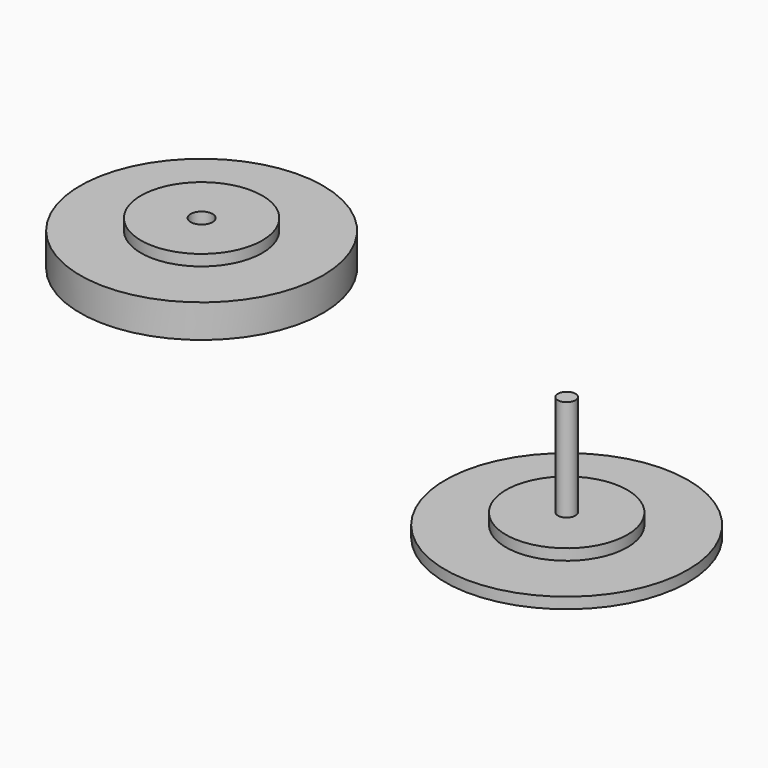
from build123d import *

# Parameters (mm, degrees)
F0_R      = 5.5
F1_DEPTH  = 0.5
F2_R      = 5.5
F3_DEPTH  = 0.5
F4_R      = 2.75
F5_DEPTH  = 1
F6_R      = 2.75
F7_DEPTH  = 1
F8_R      = 0.5
F9_DEPTH  = 0.7
F10_R     = 0.4
F11_DEPTH = 4.6
F13_DEPTH = 1


# Not quite as in the source:
# - the program builds the solid bodies; features that only make, move or delete a surface that nothing else refers to are left out


with BuildPart() as f1:
    # F0 (on Top) → F1 (new body)
    with BuildSketch(Plane.XY):
        with Locations((-49.2776818573, 41.9655069709)):
            Circle(F0_R)
    extrude(amount=F1_DEPTH)

    # F4 (on Top) → F5 (join)
    with BuildSketch(Plane.XY):
        with Locations((-49.2776595056, 41.9656410813)):
            Circle(F4_R)
    extrude(amount=F5_DEPTH)

    # F8 (on face) → F9 (cut)
    with BuildSketch(Plane.XY.offset(1)):
        with Locations((-49.2776595056, 41.9656410813)):
            Circle(F8_R)
    extrude(amount=-F9_DEPTH, mode=Mode.SUBTRACT)

    # F0 (on Top) → F13 (join)
    with BuildSketch(Plane.XY):
        with Locations((-49.2776818573, 41.9655069709)):
            Circle(F0_R)
    extrude(amount=-F13_DEPTH)


with BuildPart() as f3:
    # F2 (on Top) → F3 (new body)
    with BuildSketch(Plane.XY):
        with Locations((-25.1157227904, 32.4278958142)):
            Circle(F2_R)
    extrude(amount=F3_DEPTH)

    # F6 (on Top) → F7 (join)
    with BuildSketch(Plane.XY):
        with Locations((-25.1157619059, 32.4279852211)):
            Circle(F6_R)
    extrude(amount=F7_DEPTH)

    # F10 (on face) → F11 (join)
    with BuildSketch(Plane.XY.offset(1)):
        with Locations((-25.1157619059, 32.4279852211)):
            Circle(F10_R)
    extrude(amount=F11_DEPTH)


solid = Compound([f1.part, f3.part])
